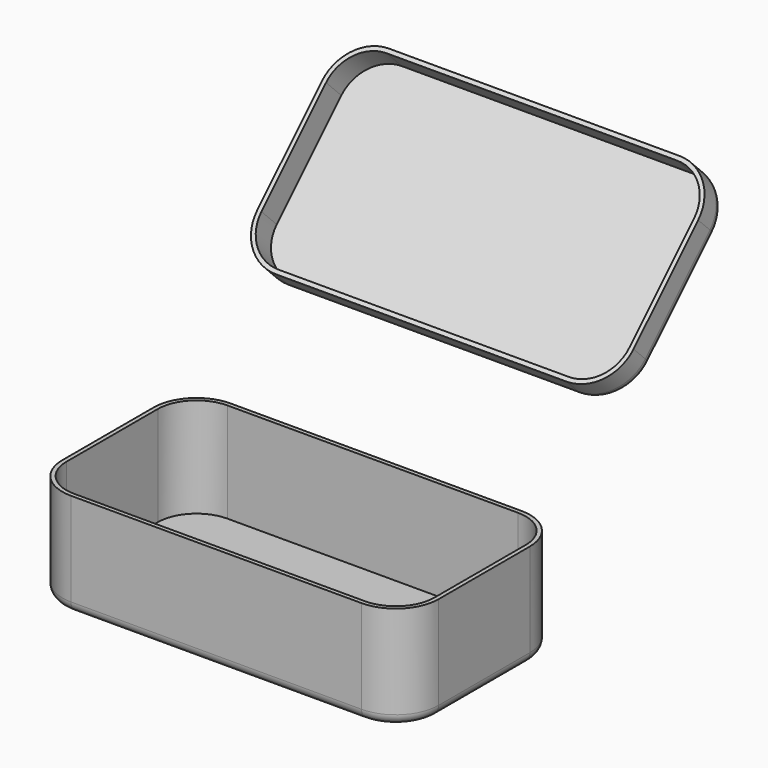
from build123d import *

# Parameters (mm, degrees)
F1_DEPTH = 50
F2_DEPTH = 2
F5_DEPTH = 2
F6_DEPTH = 15
F8_W     = 20
F8_H     = 2.4975641537
F9_DEPTH = 2
F10_R    = 5
F11_R    = 5


# Not quite as in the source:
# - a feature names something its author has since deleted; it is built from what else it names


with BuildPart() as f1:
    # F0 (on Top) → F1 (new body)
    with BuildSketch(Plane.XY):
        with BuildLine():
            ThreePointArc((-70.0215809153, 48.1610759377), (-84.5926481603, 42.1255410641), (-90.6281816654, 27.5544732523))
            Line((-90.6281816654, 27.5544732523), (-90.6281816654, -27.4455267477))
            ThreePointArc((-90.6281816654, -27.4455267477), (-84.5926486755, -42.0165950962), (-70.0215808636, -48.0521293815))
            Line((-70.0215808636, -48.0521293815), (69.9784191364, -48.0521293815))
            ThreePointArc((69.9784191364, -48.0521293815), (84.5494875406, -42.0165959566), (90.5850234457, -27.4455285797))
            Line((90.5850234457, -27.4455285797), (90.5850234457, 27.5544733039))
            ThreePointArc((90.5850234457, 27.5544733039), (84.5494881549, 42.1255418682), (69.9784190847, 48.1610759377))
            Line((69.9784190847, 48.1610759377), (-70.0215809153, 48.1610759377))
        make_face()
        with BuildLine():
            Line((69.9784191364, -46.0521293815), (-70.0215808636, -46.0521293815))
            ThreePointArc((-70.0215808636, -46.0521293815), (-83.1784344654, -40.6023821815), (-88.6281816654, -27.4455285797))
            Line((-88.6281816654, -27.4455285797), (-88.6281816654, 27.5544732523))
            ThreePointArc((-88.6281816654, 27.5544732523), (-83.1784345979, 40.7113275017), (-70.0215809153, 46.1610759377))
            Line((-70.0215809153, 46.1610759377), (69.9784190847, 46.1610759377))
            ThreePointArc((69.9784190847, 46.1610759377), (83.1352739819, 40.7113282011), (88.5850217185, 27.5544733039))
            Line((88.5850217185, 27.5544733039), (88.5850217185, -27.4455285797))
            ThreePointArc((88.5850217185, -27.4455285797), (83.1352733676, -40.6023822895), (69.9784191364, -46.0521293815))
        make_face(mode=Mode.SUBTRACT)
    extrude(amount=F1_DEPTH)

    # F0 (on Top) → F2 (join)
    with BuildSketch(Plane.XY):
        with BuildLine():
            ThreePointArc((-88.6281816654, -27.4455285797), (-83.1784344654, -40.6023821815), (-70.0215808636, -46.0521293815))
            Line((-70.0215808636, -46.0521293815), (69.9784191364, -46.0521293815))
            ThreePointArc((69.9784191364, -46.0521293815), (83.1352733676, -40.6023822895), (88.5850217185, -27.4455285797))
            Line((88.5850217185, -27.4455285797), (88.5850217185, 27.5544733039))
            ThreePointArc((88.5850217185, 27.5544733039), (83.1352739819, 40.7113282011), (69.9784190847, 46.1610759377))
            Line((69.9784190847, 46.1610759377), (-70.0215809153, 46.1610759377))
            ThreePointArc((-70.0215809153, 46.1610759377), (-83.1784345979, 40.7113275017), (-88.6281816654, 27.5544732523))
            Line((-88.6281816654, 27.5544732523), (-88.6281816654, -27.4455285797))
        make_face()
    extrude(amount=F2_DEPTH)

    # F8 (on face) → F9 (cut)
    with BuildSketch(Plane(origin=(0, 84.0832325734, 84.0832325734), x_dir=(1, 0, 0), z_dir=(0, -0.7071067812, -0.7071067812))):
        with Locations((0, -0.5405465653)):
            Rectangle(F8_W, F8_H)
    extrude(amount=-F9_DEPTH, mode=Mode.SUBTRACT)

    # F11
    f11_edges = [f1.edges().sort_by_distance(p)[0] for p in [
        (-0.021581, 48.161076, 0),
        (-84.592648, 42.125541, 0),
        (-90.628182, 0.054473, 0),
        (-84.592649, -42.016595, 0),
        (-0.021581, -48.052129, 0),
        (84.549488, -42.016596, 0),
        (90.585023, 0.054472, 0),
        (84.549488, 42.125542, 0),
    ]]
    fillet(f11_edges, radius=F11_R)


with BuildPart() as f5:
    # F4 (on face) → F5 (new body)
    with BuildSketch(Plane(origin=(0, -0.9194620312, 0.9194620312), x_dir=(1, 0, 0), z_dir=(0, -0.7071067812, 0.7071067812))):
        with BuildLine():
            ThreePointArc((-86.3849869775, 139.5182486753), (-80.9352397774, 126.3613950735), (-67.7783861756, 120.9116478734))
            Line((-67.7783861756, 120.9116478734), (72.2216138244, 120.9116478734))
            ThreePointArc((72.2216138244, 120.9116478734), (85.3784680556, 126.3613949655), (90.8282164065, 139.5182486753))
            Line((90.8282164065, 139.5182486753), (90.8282164065, 194.5182505589))
            ThreePointArc((90.8282164065, 194.5182505589), (85.3784686699, 207.675105456), (72.2216137727, 213.1248531926))
            Line((72.2216137727, 213.1248531926), (-67.7783862273, 213.1248531926))
            ThreePointArc((-67.7783862273, 213.1248531926), (-80.93523991, 207.6751047567), (-86.3849869775, 194.5182505072))
            Line((-86.3849869775, 194.5182505072), (-86.3849869775, 139.5182486753))
        make_face()
    extrude(amount=F5_DEPTH)

    # F4 (on face) → F6 (join)
    with BuildSketch(Plane(origin=(0, -0.9194620312, 0.9194620312), x_dir=(1, 0, 0), z_dir=(0, -0.7071067812, 0.7071067812))):
        with BuildLine():
            ThreePointArc((-67.7783862273, 215.1248531926), (-82.3494534723, 209.0893183191), (-88.3849869775, 194.5182505072))
            Line((-88.3849869775, 194.5182505072), (-88.3849869775, 139.5182505072))
            ThreePointArc((-88.3849869775, 139.5182505072), (-82.3494539875, 124.9471821588), (-67.7783861756, 118.9116478734))
            Line((-67.7783861756, 118.9116478734), (72.2216138244, 118.9116478734))
            ThreePointArc((72.2216138244, 118.9116478734), (86.7926822286, 124.9471812983), (92.8282181337, 139.5182486753))
            Line((92.8282181337, 139.5182486753), (92.8282181337, 194.5182505589))
            ThreePointArc((92.8282181337, 194.5182505589), (86.7926828429, 209.0893191232), (72.2216137727, 215.1248531926))
            Line((72.2216137727, 215.1248531926), (-67.7783862273, 215.1248531926))
        make_face()
        with BuildLine():
            Line((72.2216138244, 120.9116478734), (-67.7783861756, 120.9116478734))
            ThreePointArc((-67.7783861756, 120.9116478734), (-80.9352397774, 126.3613950735), (-86.3849869775, 139.5182486753))
            Line((-86.3849869775, 139.5182486753), (-86.3849869775, 194.5182505072))
            ThreePointArc((-86.3849869775, 194.5182505072), (-80.93523991, 207.6751047567), (-67.7783862273, 213.1248531926))
            Line((-67.7783862273, 213.1248531926), (72.2216137727, 213.1248531926))
            ThreePointArc((72.2216137727, 213.1248531926), (85.3784686699, 207.675105456), (90.8282164065, 194.5182505589))
            Line((90.8282164065, 194.5182505589), (90.8282164065, 139.5182486753))
            ThreePointArc((90.8282164065, 139.5182486753), (85.3784680556, 126.3613949655), (72.2216138244, 120.9116478734))
        make_face(mode=Mode.SUBTRACT)
    extrude(amount=F6_DEPTH)

    # F10
    f10_edges = [f5.edges().sort_by_distance(p)[0] for p in [
        (-82.349453, 146.929013, 148.767937),
        (-88.384987, 117.180275, 119.0192),
        (-82.349454, 87.431538, 89.270462),
        (2.221614, 83.163771, 85.002695),
        (86.792682, 87.431537, 89.270461),
        (92.828218, 117.180275, 119.019199),
        (86.792683, 146.929013, 148.767937),
        (2.221614, 151.19678, 153.035705),
    ]]
    fillet(f10_edges, radius=F10_R)


solid = Compound([f1.part, f5.part])
